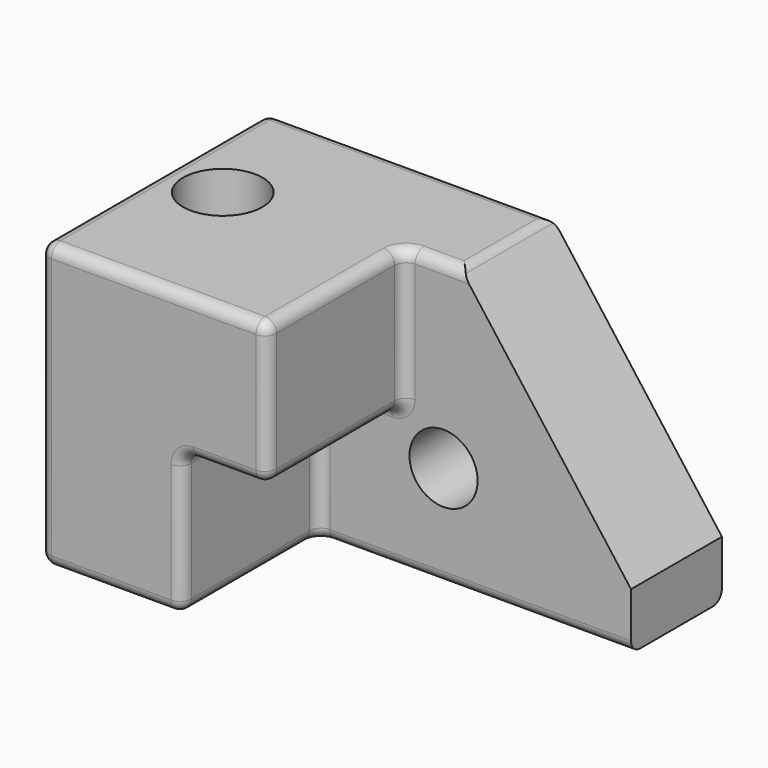
from build123d import *

# Parameters (mm, degrees)
F0_W     = 203.2
F0_H     = 127
F1_DEPTH = 127
F3_DEPTH = 76.2
F4_SIZE2 = 101.6
F4_SIZE  = 76.2
F5_R     = 5.08
F6_R     = 15.24
F7_DEPTH = 50.801
F8_R     = 17.78
F9_DEPTH = 127.001


with BuildPart() as f1:
    # F0 (on Front) → F1 (new body)
    with BuildSketch(Plane.XZ):
        Rectangle(F0_W, F0_H)
    extrude(amount=F1_DEPTH)

    # F2 (on face) → F3 (cut)
    with BuildSketch(Plane.XZ.offset(127)):
        Polygon((-38.1, 0), (-38.1, -63.5), (101.6, -63.5), (101.6, 63.5), (0, 63.5), (0, 0), align=None)
    extrude(amount=-F3_DEPTH, mode=Mode.SUBTRACT)

    # F4
    f4_edges = [f1.edges().sort_by_distance(p)[0] for p in [
        (101.6, -25.4, 63.5),
    ]]
    f4_side = f1.faces().sort_by_distance((-21.771429, -52.614286, 63.5))[0]
    chamfer(f4_edges, length=F4_SIZE, length2=F4_SIZE2, reference=f4_side)

    # F5
    f5_edges = [f1.edges().sort_by_distance(p)[0] for p in [
        (0, -127, 31.75),
        (-19.05, -127, 0),
        (-38.1, -127, -31.75),
        (-69.85, -127, -63.5),
        (-101.6, -127, 0),
        (-50.8, -127, 63.5),
        (0, -88.9, 63.5),
        (0, -88.9, 0),
        (0, -50.8, 31.75),
        (-38.1, -88.9, 0),
        (-38.1, -88.9, -63.5),
        (-38.1, -50.8, -31.75),
        (-38.1, 0, 63.5),
        (25.4, -25.4, 63.5),
        (-101.6, -63.5, 63.5),
        (12.7, -50.8, 63.5),
        (-101.6, -63.5, -63.5),
        (-101.6, 0, 0),
        (0, 0, -63.5),
        (31.75, -50.8, -63.5),
        (-19.05, -50.8, 0),
    ]]
    fillet(f5_edges, radius=F5_R)

    # F6 (on face) → F7 (cut, through all)
    with BuildSketch(Plane.XZ.offset(50.8)):
        with Locations((17.78, -17.78)):
            Circle(F6_R)
    extrude(amount=-F7_DEPTH, mode=Mode.SUBTRACT)

    # F8 (on face) → F9 (cut, through all)
    with BuildSketch(Plane.XY.offset(63.5)):
        with Locations((-75.203537941, -57.9331703484)):
            Circle(F8_R)
    extrude(amount=-F9_DEPTH, mode=Mode.SUBTRACT)


solid = f1.part
